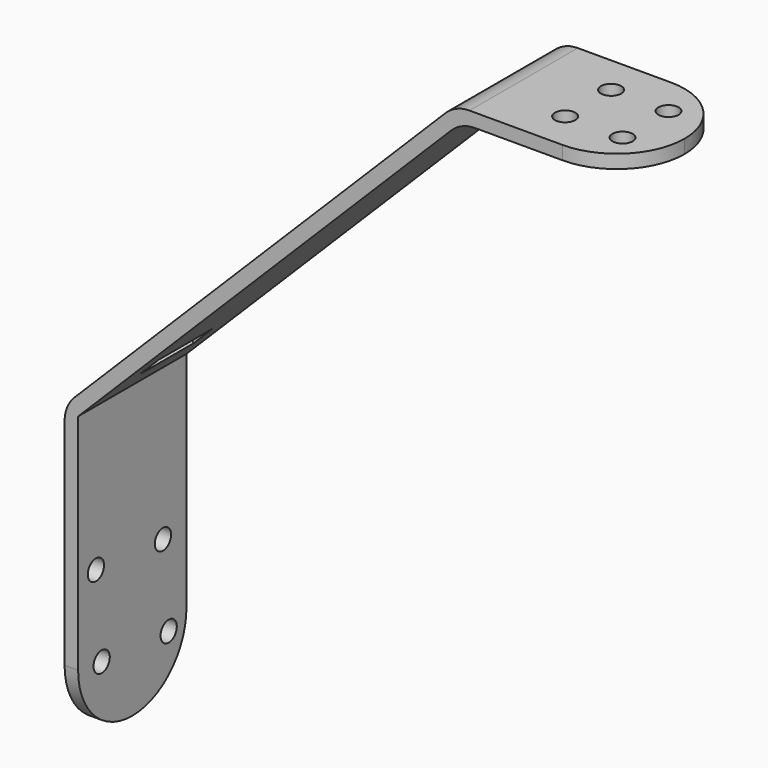
from build123d import *

# Parameters (mm, degrees)
F1_DEPTH = 20
F3_R     = 9.99999
F4_D     = 3
F5_R     = 5
F7_D     = 3
F8_W     = 4
F8_H     = 10
F9_DEPTH = 25


# Not quite as in the source:
# - a fillet or chamfer is up to 0.001 mm smaller than in the source, because OpenCascade refuses the exact size


with BuildPart() as f1:
    # F0 (on Front) → F1 (new body)
    with BuildSketch(Plane.XZ):
        Polygon((-2, 0), (0, 0), (0, 43), (56.5685424949, 99.5685424949), (81.5685424949, 99.5685424949), (81.5685424949, 101.5685424949), (55.7401153702, 101.5685424949), (-2, 43.8284271247), align=None)
    extrude(amount=F1_DEPTH)

    # F3 (radius 10 in the source; OpenCascade refuses exactly that, so slightly less here)
    f3_edges = [f1.edges().sort_by_distance(p)[0] for p in [
        (-1, -20, 0),
        (-1, 0, 0),
        (81.568542, 0, 100.568542),
        (81.568542, -20, 100.568542),
    ]]
    fillet(f3_edges, radius=F3_R)

    # F4 (through all)
    with Locations(Plane(origin=(0, 0, 99.5685424949), x_dir=(1, 0, 0), z_dir=(0, 0, -1))):
        with Locations((75.811183182, 14.2426406871), (67.3259018078, 14.2426406871), (67.3259018078, 5.7573593129), (75.811183182, 5.7573593129)):
            Hole(F4_D / 2)

    # F5
    f5_edges = [f1.edges().sort_by_distance(p)[0] for p in [
        (55.740115, -10, 101.568542),
        (56.568542, -10, 99.568542),
        (-2, -10, 43.828427),
    ]]
    fillet(f5_edges, radius=F5_R)

    # F7 (through all)
    with Locations(Plane.YZ):
        with Locations((-4.3431457505, 20.6568542495), (-16.7175144213, 21.7175144213), (-15.6568542495, 9.3431457505), (-3.2824855787, 8.2824855787)):
            Hole(F7_D / 2)

    # F8 (on face) → F9 (cut)
    with BuildSketch(Plane(origin=(-21.5, 0, 21.5), x_dir=(0.7071067812, 0, 0.7071067812), z_dir=(0.7071067812, 0, -0.7071067812))):
        with Locations((39.5918783247, 10)):
            Rectangle(F8_W, F8_H)
    extrude(amount=-F9_DEPTH, mode=Mode.SUBTRACT)


solid = f1.part
